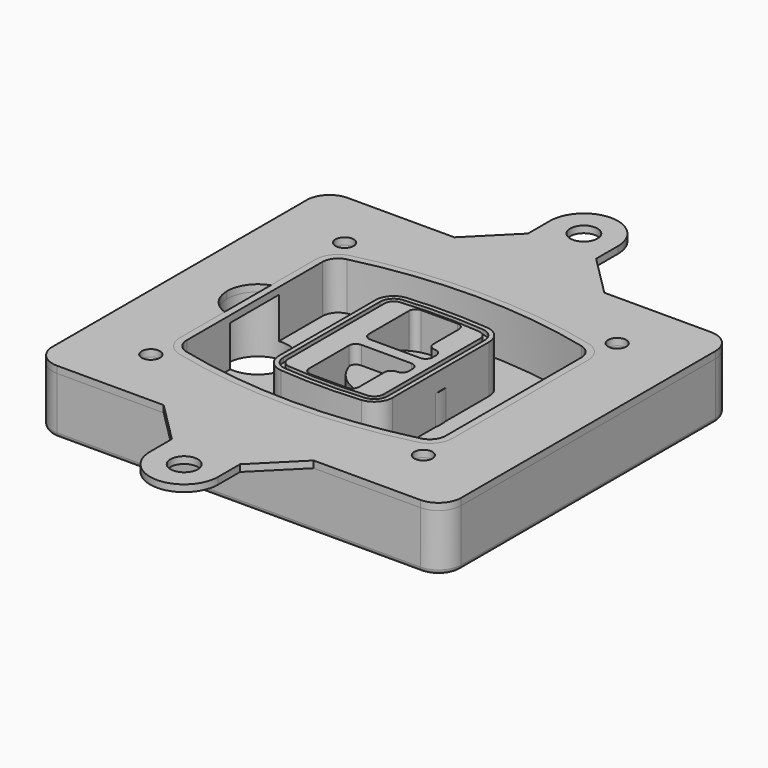
from build123d import *

# Parameters (mm, degrees)
F0_R      = 4
F1_DEPTH  = 25
F2_DEPTH  = 3
F3_DEPTH  = 18
F5_DEPTH  = 21
F6_DEPTH  = 2
F8_DEPTH  = 20
F9_DEPTH  = 16
F10_DEPTH = 25
F7_R      = 6
F7_R_2    = 4
F11_DEPTH = 6
F13_DEPTH = 9
F15_R     = 2
F16_R     = 4
F16_R_2   = 6
F17_DEPTH = 3


# Not quite as in the source:
# - a feature of the source that left no trace in its solid (it failed there, or was rolled back) is left out
# - a feature names something its author has since deleted; it is built from what else it names


with BuildPart() as f1:
    # F0 (on Top) → F1 (new body)
    with BuildSketch(Plane.XY):
        with BuildLine():
            ThreePointArc((-90, -70), (-87.0710678119, -77.0710678119), (-80, -80))
            Line((-80, -80), (80, -80))
            ThreePointArc((80, -80), (87.0710678119, -77.0710678119), (90, -70))
            Line((90, -70), (90, 70))
            ThreePointArc((90, 70), (87.0710678119, 77.0710678119), (80, 80))
            Line((80, 80), (-80, 80))
            ThreePointArc((-80, 80), (-87.0710678119, 77.0710678119), (-90, 70))
            Line((-90, 70), (-90, -70))
        make_face()
        with Locations((-60, -53.3333333333)):
            Circle(F0_R, mode=Mode.SUBTRACT)
        with Locations((60, -53.3333333333)):
            Circle(F0_R, mode=Mode.SUBTRACT)
        with Locations((-60, 53.3333333333)):
            Circle(F0_R, mode=Mode.SUBTRACT)
        with BuildLine():
            ThreePointArc((-64, 37.2990447398), (-61.0143011354, 45.9411029726), (-53.3306899286, 50.8970778549))
            ThreePointArc((-53.3306899286, 50.8970778549), (0, 57.3333333333), (53.3306899286, 50.8970778549))
            ThreePointArc((53.3306899286, 50.8970778549), (61.0143011354, 45.9411029726), (64, 37.2990447398))
            Line((64, 37.2990447398), (64, -37.2990447398))
            ThreePointArc((64, -37.2990447398), (61.0143011354, -45.9411029726), (53.3306899286, -50.8970778549))
            ThreePointArc((53.3306899286, -50.8970778549), (0, -57.3333333333), (-53.3306899286, -50.8970778549))
            ThreePointArc((-53.3306899286, -50.8970778549), (-61.0143011354, -45.9411029726), (-64, -37.2990447398))
            Line((-64, -37.2990447398), (-64, 37.2990447398))
        make_face(mode=Mode.SUBTRACT)
        with Locations((60, 53.3333333333)):
            Circle(F0_R, mode=Mode.SUBTRACT)
        with BuildLine():
            ThreePointArc((53.3306899286, 50.8970778549), (0, 57.3333333333), (-53.3306899286, 50.8970778549))
            ThreePointArc((-53.3306899286, 50.8970778549), (-61.0143011354, 45.9411029726), (-64, 37.2990447398))
            Line((-64, 37.2990447398), (-64, -37.2990447398))
            ThreePointArc((-64, -37.2990447398), (-61.0143011354, -45.9411029726), (-53.3306899286, -50.8970778549))
            ThreePointArc((-53.3306899286, -50.8970778549), (0, -57.3333333333), (53.3306899286, -50.8970778549))
            ThreePointArc((53.3306899286, -50.8970778549), (61.0143011354, -45.9411029726), (64, -37.2990447398))
            Line((64, -37.2990447398), (64, 37.2990447398))
            ThreePointArc((64, 37.2990447398), (61.0143011354, 45.9411029726), (53.3306899286, 50.8970778549))
        make_face()
        with BuildLine():
            Line((-60, -37.2990447398), (-60, 37.2990447398))
            ThreePointArc((-60, 37.2990447398), (-57.8673579538, 43.4719434775), (-52.3790642347, 47.0119255363))
            ThreePointArc((-52.3790642347, 47.0119255363), (0, 53.3333333333), (52.3790642347, 47.0119255363))
            ThreePointArc((52.3790642347, 47.0119255363), (57.8673579538, 43.4719434775), (60, 37.2990447398))
            Line((60, 37.2990447398), (60, -37.2990447398))
            ThreePointArc((60, -37.2990447398), (57.8673579538, -43.4719434775), (52.3790642347, -47.0119255363))
            ThreePointArc((52.3790642347, -47.0119255363), (0, -53.3333333333), (-52.3790642347, -47.0119255363))
            ThreePointArc((-52.3790642347, -47.0119255363), (-57.8673579538, -43.4719434775), (-60, -37.2990447398))
        make_face(mode=Mode.SUBTRACT)
        with BuildLine():
            ThreePointArc((-52.3790642347, 47.0119255363), (-57.8673579538, 43.4719434775), (-60, 37.2990447398))
            Line((-60, 37.2990447398), (-60, -37.2990447398))
            ThreePointArc((-60, -37.2990447398), (-57.8673579538, -43.4719434775), (-52.3790642347, -47.0119255363))
            ThreePointArc((-52.3790642347, -47.0119255363), (0, -53.3333333333), (52.3790642347, -47.0119255363))
            ThreePointArc((52.3790642347, -47.0119255363), (57.8673579538, -43.4719434775), (60, -37.2990447398))
            Line((60, -37.2990447398), (60, 37.2990447398))
            ThreePointArc((60, 37.2990447398), (57.8673579538, 43.4719434775), (52.3790642347, 47.0119255363))
            ThreePointArc((52.3790642347, 47.0119255363), (0, 53.3333333333), (-52.3790642347, 47.0119255363))
        make_face()
        with BuildLine():
            ThreePointArc((51.6653449643, 44.0980612973), (55.5071505677, 41.6200738562), (57, 37.2990447398))
            Line((57, 37.2990447398), (57, -37.2990447398))
            ThreePointArc((57, -37.2990447398), (55.5071505677, -41.6200738562), (51.6653449643, -44.0980612973))
            ThreePointArc((51.6653449643, -44.0980612973), (0, -50.3333333333), (-51.6653449643, -44.0980612973))
            ThreePointArc((-51.6653449643, -44.0980612973), (-55.5071505677, -41.6200738562), (-57, -37.2990447398))
            Line((-57, -37.2990447398), (-57, 37.2990447398))
            ThreePointArc((-57, 37.2990447398), (-55.5071505677, 41.6200738562), (-51.6653449643, 44.0980612973))
            ThreePointArc((-51.6653449643, 44.0980612973), (0, 50.3333333333), (51.6653449643, 44.0980612973))
        make_face(mode=Mode.SUBTRACT)
        with BuildLine():
            Line((57, -37.2990447398), (57, 37.2990447398))
            ThreePointArc((57, 37.2990447398), (55.5071505677, 41.6200738562), (51.6653449643, 44.0980612973))
            ThreePointArc((51.6653449643, 44.0980612973), (0, 50.3333333333), (-51.6653449643, 44.0980612973))
            ThreePointArc((-51.6653449643, 44.0980612973), (-55.5071505677, 41.6200738562), (-57, 37.2990447398))
            Line((-57, 37.2990447398), (-57, -37.2990447398))
            ThreePointArc((-57, -37.2990447398), (-55.5071505677, -41.6200738562), (-51.6653449643, -44.0980612973))
            ThreePointArc((-51.6653449643, -44.0980612973), (0, -50.3333333333), (51.6653449643, -44.0980612973))
            ThreePointArc((51.6653449643, -44.0980612973), (55.5071505677, -41.6200738562), (57, -37.2990447398))
        make_face()
    extrude(amount=-F1_DEPTH)

    # F0 (on Top) → F2 (join)
    with BuildSketch(Plane.XY):
        with BuildLine():
            ThreePointArc((-52.3790642347, 47.0119255363), (-57.8673579538, 43.4719434775), (-60, 37.2990447398))
            Line((-60, 37.2990447398), (-60, -37.2990447398))
            ThreePointArc((-60, -37.2990447398), (-57.8673579538, -43.4719434775), (-52.3790642347, -47.0119255363))
            ThreePointArc((-52.3790642347, -47.0119255363), (0, -53.3333333333), (52.3790642347, -47.0119255363))
            ThreePointArc((52.3790642347, -47.0119255363), (57.8673579538, -43.4719434775), (60, -37.2990447398))
            Line((60, -37.2990447398), (60, 37.2990447398))
            ThreePointArc((60, 37.2990447398), (57.8673579538, 43.4719434775), (52.3790642347, 47.0119255363))
            ThreePointArc((52.3790642347, 47.0119255363), (0, 53.3333333333), (-52.3790642347, 47.0119255363))
        make_face()
        with BuildLine():
            ThreePointArc((51.6653449643, 44.0980612973), (55.5071505677, 41.6200738562), (57, 37.2990447398))
            Line((57, 37.2990447398), (57, -37.2990447398))
            ThreePointArc((57, -37.2990447398), (55.5071505677, -41.6200738562), (51.6653449643, -44.0980612973))
            ThreePointArc((51.6653449643, -44.0980612973), (0, -50.3333333333), (-51.6653449643, -44.0980612973))
            ThreePointArc((-51.6653449643, -44.0980612973), (-55.5071505677, -41.6200738562), (-57, -37.2990447398))
            Line((-57, -37.2990447398), (-57, 37.2990447398))
            ThreePointArc((-57, 37.2990447398), (-55.5071505677, 41.6200738562), (-51.6653449643, 44.0980612973))
            ThreePointArc((-51.6653449643, 44.0980612973), (0, 50.3333333333), (51.6653449643, 44.0980612973))
        make_face(mode=Mode.SUBTRACT)
    extrude(amount=F2_DEPTH)

    # F0 (on Top) → F3 (cut)
    with BuildSketch(Plane.XY):
        with BuildLine():
            Line((57, -37.2990447398), (57, 37.2990447398))
            ThreePointArc((57, 37.2990447398), (55.5071505677, 41.6200738562), (51.6653449643, 44.0980612973))
            ThreePointArc((51.6653449643, 44.0980612973), (0, 50.3333333333), (-51.6653449643, 44.0980612973))
            ThreePointArc((-51.6653449643, 44.0980612973), (-55.5071505677, 41.6200738562), (-57, 37.2990447398))
            Line((-57, 37.2990447398), (-57, -37.2990447398))
            ThreePointArc((-57, -37.2990447398), (-55.5071505677, -41.6200738562), (-51.6653449643, -44.0980612973))
            ThreePointArc((-51.6653449643, -44.0980612973), (0, -50.3333333333), (51.6653449643, -44.0980612973))
            ThreePointArc((51.6653449643, -44.0980612973), (55.5071505677, -41.6200738562), (57, -37.2990447398))
        make_face()
    extrude(amount=-F3_DEPTH, mode=Mode.SUBTRACT)

    # F4 (on face) → F5 (join, through all)
    with BuildSketch(Plane.XY.offset(3)):
        with BuildLine():
            ThreePointArc((-25, -26.587695628), (-22.8992979869, -31.9912392117), (-17.7004291845, -34.5569740744))
            ThreePointArc((-17.7004291845, -34.5569740744), (0, -35.3333333333), (17.7004291845, -34.5569740744))
            ThreePointArc((17.7004291845, -34.5569740744), (22.8992979869, -31.9912392117), (25, -26.587695628))
            Line((25, -26.587695628), (25, 26.587695628))
            ThreePointArc((25, 26.587695628), (22.8992979869, 31.9912392117), (17.7004291845, 34.5569740744))
            ThreePointArc((17.7004291845, 34.5569740744), (0, 35.3333333333), (-17.7004291845, 34.5569740744))
            ThreePointArc((-17.7004291845, 34.5569740744), (-22.8992979869, 31.9912392117), (-25, 26.587695628))
            Line((-25, 26.587695628), (-25, -26.587695628))
        make_face()
        with BuildLine():
            ThreePointArc((17.5253218884, 32.5646544628), (21.4244734902, 30.6403533158), (23, 26.587695628))
            Line((23, 26.587695628), (23, -26.587695628))
            ThreePointArc((23, -26.587695628), (21.4244734902, -30.6403533158), (17.5253218884, -32.5646544628))
            ThreePointArc((17.5253218884, -32.5646544628), (0, -33.3333333333), (-17.5253218884, -32.5646544628))
            ThreePointArc((-17.5253218884, -32.5646544628), (-21.4244734902, -30.6403533158), (-23, -26.587695628))
            Line((-23, -26.587695628), (-23, 26.587695628))
            ThreePointArc((-23, 26.587695628), (-21.4244734902, 30.6403533158), (-17.5253218884, 32.5646544628))
            ThreePointArc((-17.5253218884, 32.5646544628), (0, 33.3333333333), (17.5253218884, 32.5646544628))
        make_face(mode=Mode.SUBTRACT)
        with BuildLine():
            Line((23, -26.587695628), (23, 26.587695628))
            ThreePointArc((23, 26.587695628), (21.4244734902, 30.6403533158), (17.5253218884, 32.5646544628))
            ThreePointArc((17.5253218884, 32.5646544628), (0, 33.3333333333), (-17.5253218884, 32.5646544628))
            ThreePointArc((-17.5253218884, 32.5646544628), (-21.4244734902, 30.6403533158), (-23, 26.587695628))
            Line((-23, 26.587695628), (-23, -26.587695628))
            ThreePointArc((-23, -26.587695628), (-21.4244734902, -30.6403533158), (-17.5253218884, -32.5646544628))
            ThreePointArc((-17.5253218884, -32.5646544628), (0, -33.3333333333), (17.5253218884, -32.5646544628))
            ThreePointArc((17.5253218884, -32.5646544628), (21.4244734902, -30.6403533158), (23, -26.587695628))
        make_face()
        with BuildLine():
            ThreePointArc((17.3502145923, 30.5723348512), (19.9496489934, 29.2894674198), (21, 26.587695628))
            Line((21, 26.587695628), (21, -26.587695628))
            ThreePointArc((21, -26.587695628), (19.9496489934, -29.2894674198), (17.3502145923, -30.5723348512))
            ThreePointArc((17.3502145923, -30.5723348512), (0, -31.3333333333), (-17.3502145923, -30.5723348512))
            ThreePointArc((-17.3502145923, -30.5723348512), (-19.9496489934, -29.2894674198), (-21, -26.587695628))
            Line((-21, -26.587695628), (-21, 26.587695628))
            ThreePointArc((-21, 26.587695628), (-19.9496489934, 29.2894674198), (-17.3502145923, 30.5723348512))
            ThreePointArc((-17.3502145923, 30.5723348512), (0, 31.3333333333), (17.3502145923, 30.5723348512))
        make_face(mode=Mode.SUBTRACT)
        with BuildLine():
            Line((21, -26.587695628), (21, 26.587695628))
            ThreePointArc((21, 26.587695628), (19.9496489934, 29.2894674198), (17.3502145923, 30.5723348512))
            ThreePointArc((17.3502145923, 30.5723348512), (0, 31.3333333333), (-17.3502145923, 30.5723348512))
            ThreePointArc((-17.3502145923, 30.5723348512), (-19.9496489934, 29.2894674198), (-21, 26.587695628))
            Line((-21, 26.587695628), (-21, -26.587695628))
            ThreePointArc((-21, -26.587695628), (-19.9496489934, -29.2894674198), (-17.3502145923, -30.5723348512))
            ThreePointArc((-17.3502145923, -30.5723348512), (0, -31.3333333333), (17.3502145923, -30.5723348512))
            ThreePointArc((17.3502145923, -30.5723348512), (19.9496489934, -29.2894674198), (21, -26.587695628))
        make_face()
        with BuildLine():
            Line((-8, -2.5), (14, -2.5))
            ThreePointArc((14, -2.5), (16.1213203436, -3.3786796564), (17, -5.5))
            Line((17, -5.5), (17, -7.5))
            ThreePointArc((17, -7.5), (16.1213203436, -9.6213203436), (14, -10.5))
            ThreePointArc((14, -10.5), (11.8786796564, -11.3786796564), (11, -13.5))
            Line((11, -13.5), (11, -27.5))
            ThreePointArc((11, -27.5), (10.1213203436, -29.6213203436), (8, -30.5))
            Line((8, -30.5), (-8, -30.5))
            ThreePointArc((-8, -30.5), (-10.1213203436, -29.6213203436), (-11, -27.5))
            Line((-11, -27.5), (-11, -5.5))
            ThreePointArc((-11, -5.5), (-10.1213203436, -3.3786796564), (-8, -2.5))
        make_face(mode=Mode.SUBTRACT)
        with BuildLine():
            ThreePointArc((-8, 2.5), (-10.1213203436, 3.3786796564), (-11, 5.5))
            Line((-11, 5.5), (-11, 27.5))
            ThreePointArc((-11, 27.5), (-10.1213203436, 29.6213203436), (-8, 30.5))
            Line((-8, 30.5), (8, 30.5))
            ThreePointArc((8, 30.5), (10.1213203436, 29.6213203436), (11, 27.5))
            Line((11, 27.5), (11, 13.5))
            ThreePointArc((11, 13.5), (11.8786796564, 11.3786796564), (14, 10.5))
            ThreePointArc((14, 10.5), (16.1213203436, 9.6213203436), (17, 7.5))
            Line((17, 7.5), (17, 5.5))
            ThreePointArc((17, 5.5), (16.1213203436, 3.3786796564), (14, 2.5))
            Line((14, 2.5), (-8, 2.5))
        make_face(mode=Mode.SUBTRACT)
    extrude(amount=-F5_DEPTH)

    # F4 (on face) → F6 (cut)
    with BuildSketch(Plane.XY.offset(3)):
        with BuildLine():
            Line((23, -26.587695628), (23, 26.587695628))
            ThreePointArc((23, 26.587695628), (21.4244734902, 30.6403533158), (17.5253218884, 32.5646544628))
            ThreePointArc((17.5253218884, 32.5646544628), (0, 33.3333333333), (-17.5253218884, 32.5646544628))
            ThreePointArc((-17.5253218884, 32.5646544628), (-21.4244734902, 30.6403533158), (-23, 26.587695628))
            Line((-23, 26.587695628), (-23, -26.587695628))
            ThreePointArc((-23, -26.587695628), (-21.4244734902, -30.6403533158), (-17.5253218884, -32.5646544628))
            ThreePointArc((-17.5253218884, -32.5646544628), (0, -33.3333333333), (17.5253218884, -32.5646544628))
            ThreePointArc((17.5253218884, -32.5646544628), (21.4244734902, -30.6403533158), (23, -26.587695628))
        make_face()
        with BuildLine():
            ThreePointArc((17.3502145923, 30.5723348512), (19.9496489934, 29.2894674198), (21, 26.587695628))
            Line((21, 26.587695628), (21, -26.587695628))
            ThreePointArc((21, -26.587695628), (19.9496489934, -29.2894674198), (17.3502145923, -30.5723348512))
            ThreePointArc((17.3502145923, -30.5723348512), (0, -31.3333333333), (-17.3502145923, -30.5723348512))
            ThreePointArc((-17.3502145923, -30.5723348512), (-19.9496489934, -29.2894674198), (-21, -26.587695628))
            Line((-21, -26.587695628), (-21, 26.587695628))
            ThreePointArc((-21, 26.587695628), (-19.9496489934, 29.2894674198), (-17.3502145923, 30.5723348512))
            ThreePointArc((-17.3502145923, 30.5723348512), (0, 31.3333333333), (17.3502145923, 30.5723348512))
        make_face(mode=Mode.SUBTRACT)
    extrude(amount=-F6_DEPTH, mode=Mode.SUBTRACT)

    # F7 (on face) → F8 (join)
    with BuildSketch(Plane(origin=(0, 0, -25), x_dir=(1, 0, 0), z_dir=(0, 0, -1))):
        with BuildLine():
            ThreePointArc((-6.71157564, 0), (6.7567035675, 13.4682792075), (20.224982775, 0))
            Line((20.224982775, 0), (25.224982775, 0))
            ThreePointArc((25.224982775, 0), (6.7567035675, 18.4682792075), (-11.71157564, 0))
            Line((-11.71157564, 0), (-6.71157564, 0))
        make_face()
        with BuildLine():
            Line((-6.71157564, 0), (20.224982775, 0))
            ThreePointArc((20.224982775, 0), (6.7567035675, 13.4682792075), (-6.71157564, 0))
        make_face()
        with BuildLine():
            ThreePointArc((-6.71157564, 0), (6.7567035675, -13.4682792075), (20.224982775, 0))
            Line((20.224982775, 0), (-6.71157564, 0))
        make_face()
        with BuildLine():
            Line((25.224982775, 0), (20.224982775, 0))
            ThreePointArc((20.224982775, 0), (6.7567035675, -13.4682792075), (-6.71157564, 0))
            Line((-6.71157564, 0), (-11.71157564, 0))
            ThreePointArc((-11.71157564, 0), (6.7567035675, -18.4682792075), (25.224982775, 0))
        make_face()
    extrude(amount=-F8_DEPTH)

    # F7 (on face) → F9 (cut)
    with BuildSketch(Plane(origin=(0, 0, -25), x_dir=(1, 0, 0), z_dir=(0, 0, -1))):
        with BuildLine():
            Line((-6.71157564, 0), (20.224982775, 0))
            ThreePointArc((20.224982775, 0), (6.7567035675, 13.4682792075), (-6.71157564, 0))
        make_face()
        with BuildLine():
            ThreePointArc((-6.71157564, 0), (6.7567035675, -13.4682792075), (20.224982775, 0))
            Line((20.224982775, 0), (-6.71157564, 0))
        make_face()
    extrude(amount=-F9_DEPTH, mode=Mode.SUBTRACT)

    # F7 (on face) → F10 (cut)
    with BuildSketch(Plane(origin=(0, 0, -25), x_dir=(1, 0, 0), z_dir=(0, 0, -1))):
        with BuildLine():
            Line((-69.0318229325, 0), (-42.0952645175, 0))
            ThreePointArc((-42.0952645175, 0), (-55.563543725, 13.4682792075), (-69.0318229325, 0))
        make_face()
        with BuildLine():
            ThreePointArc((-69.0318229325, 0), (-55.563543725, -13.4682792075), (-42.0952645175, 0))
            Line((-42.0952645175, 0), (-69.0318229325, 0))
        make_face()
    extrude(amount=-F10_DEPTH, mode=Mode.SUBTRACT)

    # F7 (on face) → F11 (cut)
    with BuildSketch(Plane(origin=(0, 0, -25), x_dir=(1, 0, 0), z_dir=(0, 0, -1))):
        with Locations((60, -53.3333333333)):
            Circle(F7_R)
        with Locations((60, -53.3333333333)):
            Circle(F7_R_2, mode=Mode.SUBTRACT)
        with Locations((-60, -53.3333333333)):
            Circle(F7_R)
        with Locations((-60, -53.3333333333)):
            Circle(F7_R_2, mode=Mode.SUBTRACT)
        with Locations((-60, 53.3333333333)):
            Circle(F7_R)
        with Locations((-60, 53.3333333333)):
            Circle(F7_R_2, mode=Mode.SUBTRACT)
        with Locations((60, 53.3333333333)):
            Circle(F7_R)
        with Locations((60, 53.3333333333)):
            Circle(F7_R_2, mode=Mode.SUBTRACT)
    extrude(amount=-F11_DEPTH, mode=Mode.SUBTRACT)

    # F12 (on face) → F13 (cut, through all)
    with BuildSketch(Plane(origin=(0, 0, -9), x_dir=(1, 0, 0), z_dir=(0, 0, -1))):
        with BuildLine():
            ThreePointArc((20.224982775, 0), (20.1663399806, 1.2554664788), (19.9909222755, 2.5))
            Line((19.9909222755, 2.5), (14, 2.5))
            ThreePointArc((14, 2.5), (16.1213203436, 3.3786796564), (17, 5.5))
            Line((17, 5.5), (17, 7.5))
            ThreePointArc((17, 7.5), (16.1213203436, 9.6213203436), (14, 10.5))
            ThreePointArc((14, 10.5), (12.1627255951, 11.1284134507), (11.0951631559, 12.750384826))
            ThreePointArc((11.0951631559, 12.750384826), (11.0476113807, 12.7664660322), (11, 12.7823698976))
            Line((11, 12.7823698976), (11, -12.7823698976))
            ThreePointArc((11, -12.7823698976), (11.0476113807, -12.7664660322), (11.0951631559, -12.750384826))
            ThreePointArc((11.0951631559, -12.750384826), (12.1627255951, -11.1284134507), (14, -10.5))
            ThreePointArc((14, -10.5), (16.1213203436, -9.6213203436), (17, -7.5))
            Line((17, -7.5), (17, -5.5))
            ThreePointArc((17, -5.5), (16.1213203436, -3.3786796564), (14, -2.5))
            Line((14, -2.5), (19.9909222755, -2.5))
            ThreePointArc((19.9909222755, -2.5), (20.1663399806, -1.2554664788), (20.224982775, 0))
        make_face()
    extrude(amount=F13_DEPTH, mode=Mode.SUBTRACT)

    # F15
    f15_edges = [f1.edges().sort_by_distance(p)[0] for p in [
        (0, -80, -25),
        (-87.071068, -77.071068, -25),
        (-90, 0, -25),
        (-87.071068, 77.071068, -25),
        (87.071068, -77.071068, -25),
        (0, 80, -25),
        (90, 0, -25),
        (87.071068, 77.071068, -25),
    ]]
    fillet(f15_edges, radius=F15_R)


with BuildPart() as f17:
    # F16 (on face) → F17 (new body, through all)
    with BuildSketch(Plane.XY):
        with BuildLine():
            Line((33, 80), (-33, 80))
            Line((-33, 80), (-80, 80))
            ThreePointArc((-80, 80), (-87.0710678119, 77.0710678119), (-90, 70))
            Line((-90, 70), (-90, -70))
            ThreePointArc((-90, -70), (-87.0710678119, -77.0710678119), (-80, -80))
            Line((-80, -80), (-33, -80))
            Line((-33, -80), (33, -80))
            Line((33, -80), (80, -80))
            ThreePointArc((80, -80), (87.0710678119, -77.0710678119), (90, -70))
            Line((90, -70), (90, 70))
            ThreePointArc((90, 70), (87.0710678119, 77.0710678119), (80, 80))
            Line((80, 80), (33, 80))
        make_face()
        with Locations((-60, -53.3333333333)):
            Circle(F16_R, mode=Mode.SUBTRACT)
        with BuildLine():
            Line((-60, 12.7166190685), (-60, 37.2990447398))
            ThreePointArc((-60, 37.2990447398), (-57.8673579538, 43.4719434775), (-52.3790642347, 47.0119255363))
            ThreePointArc((-52.3790642347, 47.0119255363), (0, 53.3333333333), (52.3790642347, 47.0119255363))
            ThreePointArc((52.3790642347, 47.0119255363), (57.8673579538, 43.4719434775), (60, 37.2990447398))
            Line((60, 37.2990447398), (60, -37.2990447398))
            ThreePointArc((60, -37.2990447398), (57.8673579538, -43.4719434775), (52.3790642347, -47.0119255363))
            ThreePointArc((52.3790642347, -47.0119255363), (0, -53.3333333333), (-52.3790642347, -47.0119255363))
            ThreePointArc((-52.3790642347, -47.0119255363), (-57.8673579538, -43.4719434775), (-60, -37.2990447398))
            Line((-60, -37.2990447398), (-60, -12.7166190685))
            ThreePointArc((-60, -12.7166190685), (-66.5441169481, -7.798817635), (-69.0318229325, 0))
            ThreePointArc((-69.0318229325, 0), (-66.5441169481, 7.798817635), (-60, 12.7166190685))
        make_face(mode=Mode.SUBTRACT)
        with Locations((60, -53.3333333333)):
            Circle(F16_R, mode=Mode.SUBTRACT)
        with Locations((-60, 53.3333333333)):
            Circle(F16_R, mode=Mode.SUBTRACT)
        with Locations((60, 53.3333333333)):
            Circle(F16_R, mode=Mode.SUBTRACT)
        with BuildLine():
            ThreePointArc((15, 110), (0, 125), (-15, 110))
            Line((-15, 110), (-15, 98))
            Line((-15, 98), (-33, 80))
            Line((-33, 80), (33, 80))
            Line((33, 80), (15, 98))
            Line((15, 98), (15, 110))
        make_face()
        with Locations((0, 110)):
            Circle(F16_R_2, mode=Mode.SUBTRACT)
        with BuildLine():
            Line((33, -80), (-33, -80))
            Line((-33, -80), (-15, -98))
            Line((-15, -98), (-15, -110))
            ThreePointArc((-15, -110), (0, -125), (15, -110))
            Line((15, -110), (15, -98))
            Line((15, -98), (33, -80))
        make_face()
        with Locations((0, -110)):
            Circle(F16_R_2, mode=Mode.SUBTRACT)
    extrude(amount=F17_DEPTH)


solid = Compound([f1.part, f17.part])
